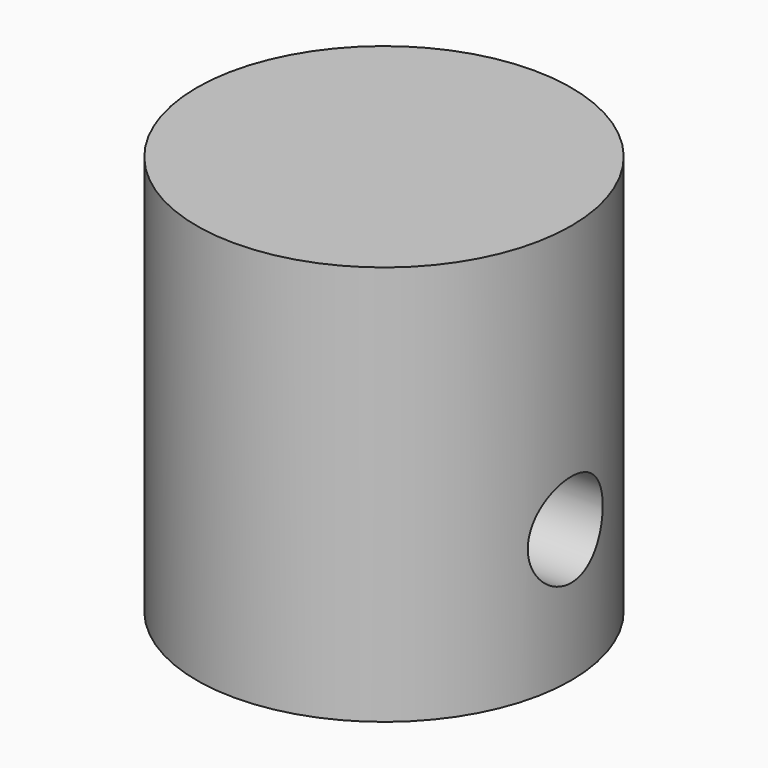
from build123d import *

# Parameters (mm, degrees)
F0_R          = 14
F1_DEPTH      = 30
F2_T          = -5
F3_R          = 3.5
F4_DEPTH      = 14.001
F4_DEPTH_BACK = 14.001


# Not quite as in the source:
# - a fillet or chamfer that OpenCascade refuses, or shapes differently, is made with other operations: its cross-section is extruded or revolved along the edge and cut away or added


with BuildPart() as f1:
    # F0 (on Top) → F1 (new body)
    with BuildSketch(Plane.XY):
        Circle(F0_R)
    extrude(amount=F1_DEPTH)

    # F2
    f2_openings = [f1.faces().sort_by_distance(p)[0] for p in [
        (0, 0, 0),
    ]]
    offset(amount=F2_T, openings=f2_openings)

    # F3 (on Right) → F4 (cut, two sides)
    with BuildSketch(Plane.YZ) as f4_sk:
        with Locations((0, 10)):
            Circle(F3_R)
    extrude(amount=-F4_DEPTH, mode=Mode.SUBTRACT)
    extrude(f4_sk.sketch, amount=F4_DEPTH_BACK, mode=Mode.SUBTRACT)

    # F5: chamfer of 5.08 on 1 edges, made by hand

    # F5_s1 → F5_t2 (revolve, cut)
    with BuildSketch(Plane.XZ):
        Polygon((14.08, 0), (9, 5.08), (9, 0), align=None)
    revolve(axis=Axis((0, 0, 0), (0, 0, 1)), mode=Mode.SUBTRACT)


solid = f1.part
